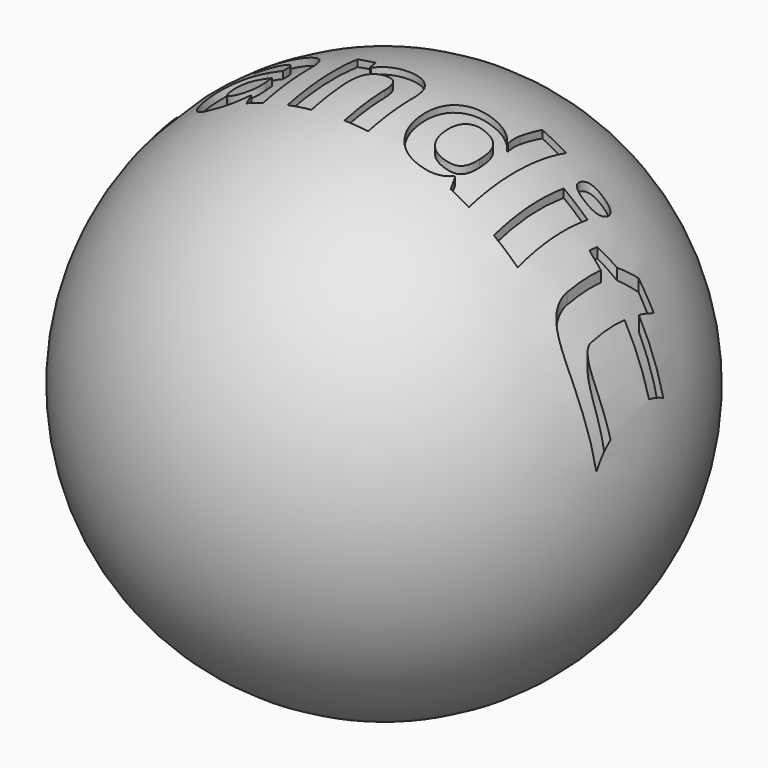
from build123d import *

# Parameters (mm, degrees)
F2_TEXT_SIZE = 30.7815890822
F3_DEPTH     = 81.28


# Not quite as in the source:
# - Text() gives the source's letters only with a copy of the font that has no kerning and outlines rounded to 1/6400 em; it was checked with that copy


with BuildPart() as f1:
    # F0 (on Front) → F1 (revolve)
    with BuildSketch(Plane.XZ):
        with BuildLine():
            Line((0, -50.8), (0, 50.8))
            ThreePointArc((0, 50.8), (-50.8, 0), (0, -50.8))
        make_face()
    revolve(axis=Axis((0, 0, 0), (0, 0, -1)))

    # F2 (on Top) → F3 (cut)
    with BuildSketch(Plane.XY):
        with Locations((-51.3715864043, -11.0813720696)):
            Text('Bandit', F2_TEXT_SIZE, font='Open Sans', font_style=FontStyle.BOLD, text_align=(TextAlign.LEFT, TextAlign.BOTTOM))
    extrude(amount=F3_DEPTH, mode=Mode.SUBTRACT)

    # F4 (on Right) → F5 (revolve)
    with BuildSketch(Plane.YZ):
        with BuildLine():
            Line((-49.53, 0), (49.53, 0))
            ThreePointArc((49.53, 0), (0, 49.53), (-49.53, 0))
        make_face()
    revolve(axis=Axis((0, 0, 0), (0, -1, 0)))


solid = f1.part
